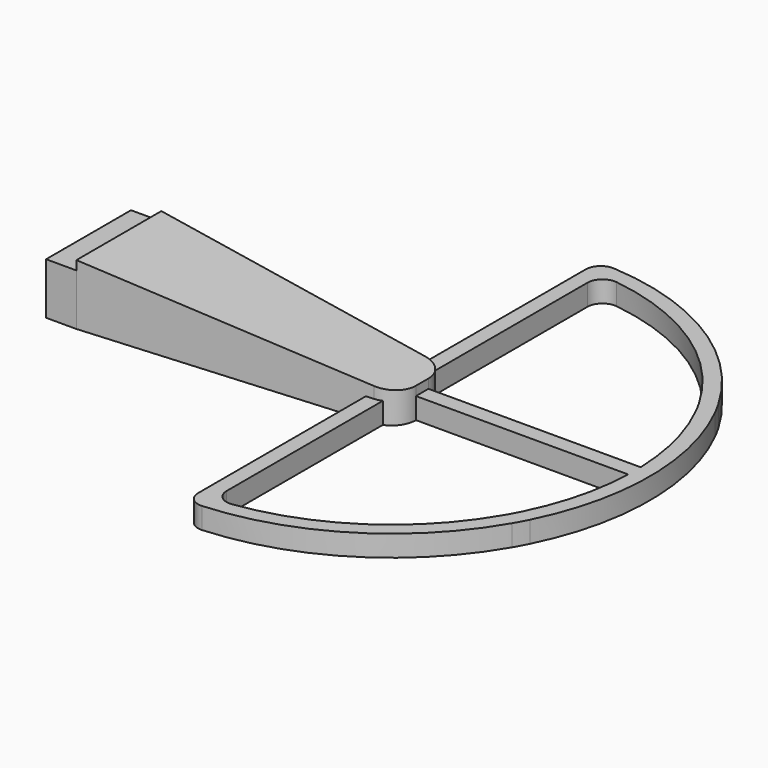
from build123d import *

# Parameters (mm, degrees)
F1_DEPTH = 10
F2_DEPTH = 17
F3_W     = 100
F3_H     = 35
F4_DEPTH = 3
F5_SIZE2 = 99.99999
F5_SIZE  = 7.49999
F6_SIZE2 = 9.99999
F6_SIZE  = 99.99999
F7_R     = 8
F9_DEPTH = 7
F10_W    = 5.1550631039
F10_H    = 7


# Not quite as in the source:
# - a fillet or chamfer is up to 0.001 mm smaller than in the source, because OpenCascade refuses the exact size
# - a feature of the source that left no trace in its solid (it failed there, or was rolled back) is left out


with BuildPart() as f1:
    # F0 (on Top) → F1 (new body)
    with BuildSketch(Plane.XY):
        Polygon((-58.5, -8.5), (-58.5, -2.5), (-58.5, 0), (-58.5, 2.5), (-58.5, 8.5), (-63.5, 0), align=None)
        Polygon((-58.5, -2.5), (-55, -2.5), (-55, 2.5), (-58.5, 2.5), (-58.5, 0), align=None)
    extrude(amount=F1_DEPTH)

    # F0 (on Top) → F2 (join)
    with BuildSketch(Plane.XY):
        Polygon((-55, -17.5), (55, -17.5), (55, 17.5), (-55, 17.5), (-55, 2.5), (-55, -2.5), align=None)
    extrude(amount=F2_DEPTH)

    # F3 (on face) → F4 (join)
    with BuildSketch(Plane.XY.offset(17)):
        with Locations((5, 0)):
            Rectangle(F3_W, F3_H)
    extrude(amount=F4_DEPTH)

    # F5 (size 7.5 and 100 in the source; OpenCascade refuses exactly that, so slightly less here)
    f5_edges = [f1.edges().sort_by_distance(p)[0] for p in [
        (55, -17.5, 10),
        (55, 17.5, 10),
    ]]
    f5_side = f1.faces().sort_by_distance((55, 0, 10))[0]
    chamfer(f5_edges, length=F5_SIZE, length2=F5_SIZE2, reference=f5_side)

    # F6 (size 100 and 10 in the source; OpenCascade refuses exactly that, so slightly less here)
    f6_edges = [f1.edges().sort_by_distance(p)[0] for p in [
        (55, 0, 20),
    ]]
    chamfer(f6_edges, length=F6_SIZE, length2=F6_SIZE2)

    # F7
    f7_edges = [f1.edges().sort_by_distance(p)[0] for p in [
        (55, -10.00001, 5.000005),
        (55, 10.00001, 5.000005),
    ]]
    fillet(f7_edges, radius=F7_R)

    # F8 (on face) → F9 (join)
    with BuildSketch(Plane.XY):
        with BuildLine():
            ThreePointArc((118.6121593217, 42.5), (89.7807277981, 72.2473973087), (50.3125, 84.8338219329))
            ThreePointArc((50.3125, 84.8338219329), (46.5767340156, 83.4879420476), (45, 79.8435971134))
            Line((45, 79.8435971134), (45, 0))
            Line((45, 0), (50, 2.8867513459))
            Line((50, 2.8867513459), (50, 74.3303437366))
            ThreePointArc((50, 74.3303437366), (51.708597057, 78.0942070001), (55.6666666667, 79.2856999857))
            ThreePointArc((55.6666666667, 79.2856999857), (89.5397594579, 66.4545696505), (114.2820323028, 40))
            Line((114.2820323028, 40), (118.6121593217, 42.5))
        make_face()
        with BuildLine():
            ThreePointArc((120.9846922835, 38.0962798523), (119.8308271392, 40.3155963576), (118.6121593217, 42.5))
            Line((118.6121593217, 42.5), (114.2820323028, 40))
            ThreePointArc((114.2820323028, 40), (115.4987732023, 37.8143223789), (116.6465834297, 35.5916715378))
            Line((116.6465834297, 35.5916715378), (120.9846922835, 38.0962798523))
        make_face()
        with BuildLine():
            ThreePointArc((120.9846922835, -38.0962798523), (130, 0), (120.9846922835, 38.0962798523))
            Line((120.9846922835, 38.0962798523), (116.6465834297, 35.5916715378))
            ThreePointArc((116.6465834297, 35.5916715378), (125, 0), (116.6465834297, -35.5916715378))
            Line((116.6465834297, -35.5916715378), (120.9846922835, -38.0962798523))
        make_face()
        with BuildLine():
            Line((50, -2.8867513459), (45, 0))
            Line((45, 0), (45, -79.8435971134))
            ThreePointArc((45, -79.8435971134), (46.5767340156, -83.4879420476), (50.3125, -84.8338219329))
            ThreePointArc((50.3125, -84.8338219329), (89.7807277981, -72.2473973087), (118.6121593217, -42.5))
            Line((118.6121593217, -42.5), (114.2820323028, -40))
            ThreePointArc((114.2820323028, -40), (89.5397594579, -66.4545696505), (55.6666666667, -79.2856999857))
            ThreePointArc((55.6666666667, -79.2856999857), (51.708597057, -78.0942070001), (50, -74.3303437366))
            Line((50, -74.3303437366), (50, -2.8867513459))
        make_face()
        Polygon((50, 2.8867513459), (45, 0), (50, -2.8867513459), align=None)
        with BuildLine():
            ThreePointArc((118.6121593217, -42.5), (119.8308271392, -40.3155963576), (120.9846922835, -38.0962798523))
            Line((120.9846922835, -38.0962798523), (116.6465834297, -35.5916715378))
            ThreePointArc((116.6465834297, -35.5916715378), (115.4987732023, -37.8143223789), (114.2820323028, -40))
            Line((114.2820323028, -40), (118.6121593217, -42.5))
        make_face()
    extrude(amount=F9_DEPTH)

    # F10 (on face) → F11 (join, up to the next surface of F1)
    with BuildSketch(Plane.YZ.offset(55)):
        with Locations((0, 3.5)):
            Rectangle(F10_W, F10_H)
    extrude(until=Until.NEXT)


solid = f1.part
